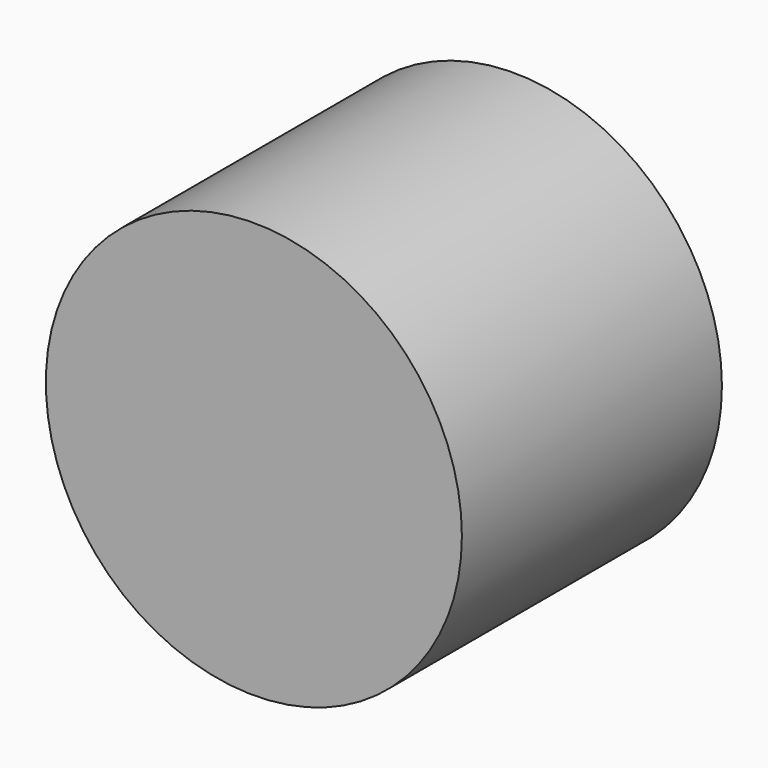
from build123d import *

# Parameters (mm, degrees)
F2_R     = 16
F3_DEPTH = 25


# Not quite as in the source:
# - the program builds the solid bodies; features that only make, move or delete a surface that nothing else refers to are left out


with BuildPart() as f3:
    # F2 (on face) → F3 (new body)
    with BuildSketch(Plane.XZ):
        with Locations((0, 44.991903007)):
            Circle(F2_R)
    extrude(amount=F3_DEPTH)


solid = f3.part
